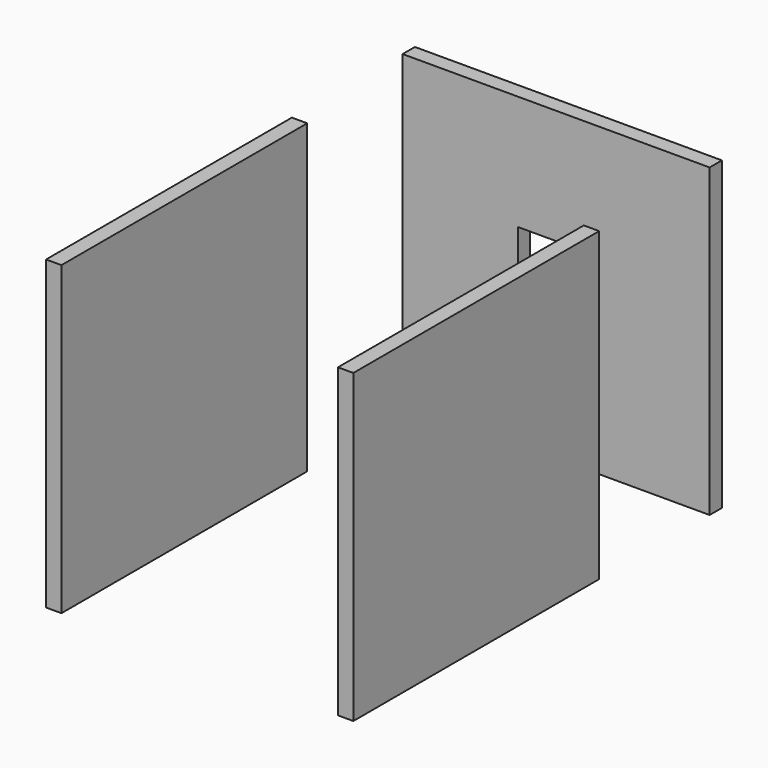
from build123d import *

# Parameters (mm, degrees)
F3_W      = 609.1041564941
F3_H      = 607.0808172226
F3_W_2    = 151.7698764801
F3_H_2    = 151.7701148987
F4_DEPTH  = 30.48
F1_E10_W  = 607.9699874166
F1_E10_H  = 609.6
F8_DEPTH  = 30.48
F11_W     = 145.6189155579
F11_H     = 147.8253602982
F12_DEPTH = 30.48


# Not quite as in the source:
# - a feature of the source that left no trace in its solid (it failed there, or was rolled back) is left out
# - a pattern or mirror of a feature is missing from the dataset's text; its kind, count and spacing are read off the source's solid
# - the program builds the solid bodies; features that only make, move or delete a surface that nothing else refers to are left out


with BuildPart() as f4:
    # F3 (on offset) → F4 (new body)
    with BuildSketch(Plane.XZ.offset(-914.4)):
        Rectangle(F3_W, F3_H)
        Rectangle(F3_W_2, F3_H_2, mode=Mode.SUBTRACT)
    extrude(amount=F4_DEPTH)


with BuildPart() as f8:
    # F1_E10 (on explicit) → F8 (new body)
    with BuildSketch(Plane(origin=(-304.8, 0, 303.9849937083), x_dir=(0, 0, -1), z_dir=(1, 0, 0))):
        with Locations((303.9849937083, 304.8)):
            Rectangle(F1_E10_W, F1_E10_H)
    extrude(amount=F8_DEPTH)


with BuildPart() as f8_copies_1:
    # F8_copies: instance of F8
    add(f8.part.mirror(Plane(origin=(0, 0, 0), x_dir=(0, 0, 1), z_dir=(1, 0, 0))))


with BuildPart() as f12:
    # F11 (on offset) → F12 (new body)
    with BuildSketch(Plane.XZ.offset(-1066.8)):
        Rectangle(F11_W, F11_H)
    extrude(amount=F12_DEPTH)


solid = Compound([f4.part, f8.part, f8_copies_1.part, f12.part])
